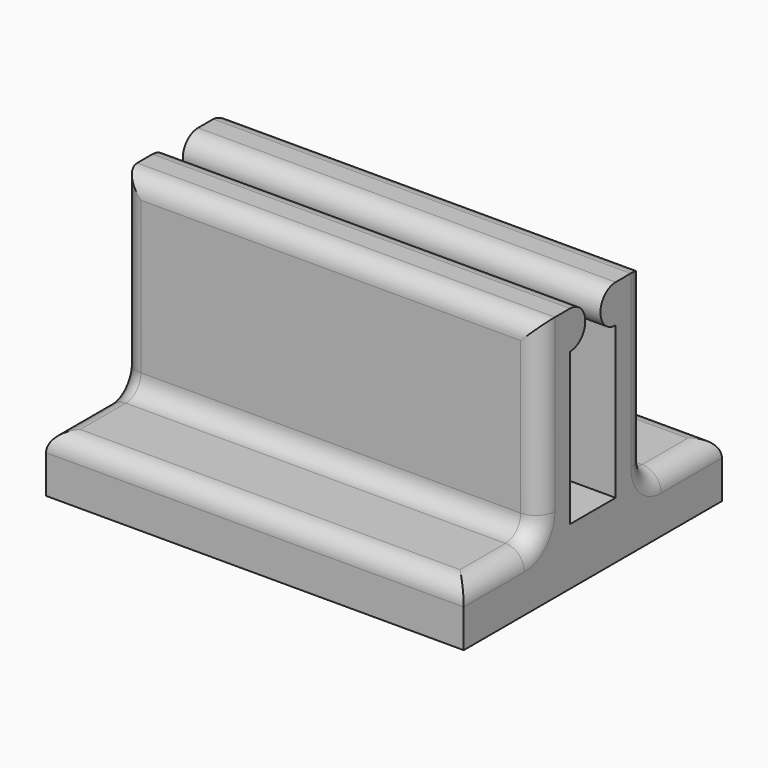
from build123d import *

# Parameters (mm, degrees)
F0_W     = 22
F0_H     = 17
F1_DEPTH = 3
F2_W     = 22
F2_H     = 2
F3_DEPTH = 10
F4_W     = 22
F4_H     = 1
F7_R     = 1


with BuildPart() as f1:
    # F0 (on Top) → F1 (new body)
    with BuildSketch(Plane.XY):
        Rectangle(F0_W, F0_H)
    extrude(amount=F1_DEPTH)

    # F2 (on face) → F3 (join)
    with BuildSketch(Plane.XY.offset(3)):
        with Locations((0, 2.5)):
            Rectangle(F2_W, F2_H)
        with Locations((0, -2.5)):
            Rectangle(F2_W, F2_H)
    extrude(amount=F3_DEPTH)

    # F4 (on face) → F5 (revolve)
    with BuildSketch(Plane.XZ.offset(-1.5)):
        with Locations((0, 12.5)):
            Rectangle(F4_W, F4_H)
    revolve(axis=Axis((0, 1.5, 12), (-1, 0, 0)))

    # F6: F1 across plane


with BuildPart() as f1_1:
    add(f1.part)
    add(f1.part.mirror(Plane.XZ))

    # F7
    f7_edges = [f1_1.edges().sort_by_distance(p)[0] for p in [
        (0, -3.5, 3),
        (0, -3.5, 13),
        (11, 3.5, 8),
        (11, -6, 3),
        (0, -8.5, 3),
        (-11, -6, 3),
        (0, 3.5, 13),
        (0, 3.5, 3),
        (-11, 6, 3),
        (11, 6, 3),
        (0, 8.5, 3),
        (-11, 3.5, 8),
        (-11, -3.5, 8),
        (11, -3.5, 8),
    ]]
    fillet(f7_edges, radius=F7_R)


solid = f1_1.part
